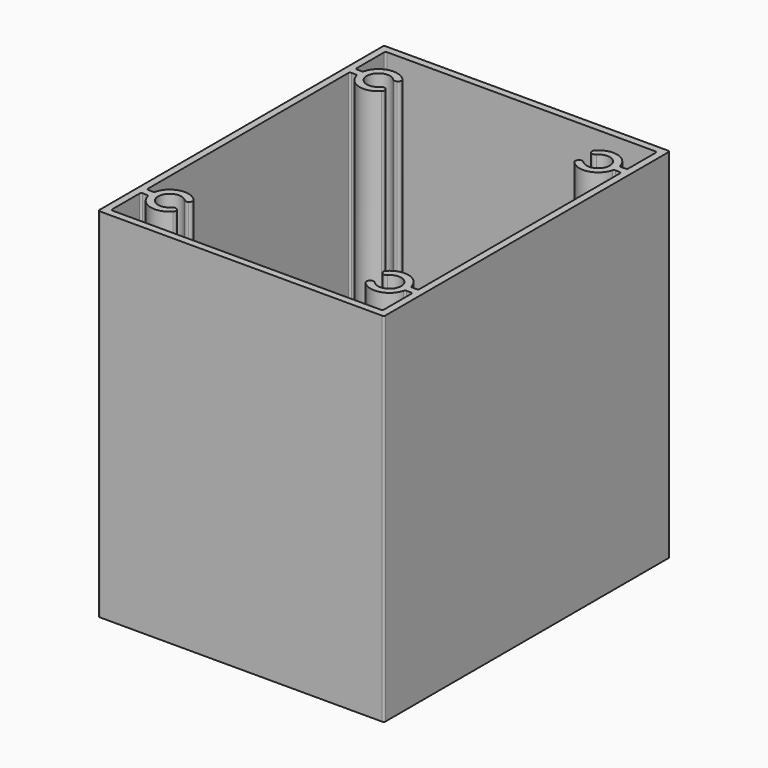
from build123d import *

# Parameters (mm, degrees)
F1_DEPTH = 100


# Not quite as in the source:
# - ends of sketch curves that miss each other by under 0.0002 mm in the source are joined


with BuildPart() as f1:
    # F0 (on Top) → F1 (new body)
    with BuildSketch(Plane.XY):
        with BuildLine():
            Line((40, -49.5), (40, 49.5))
            ThreePointArc((40, 49.5), (39.8535533906, 49.8535533906), (39.5, 50))
            Line((39.5, 50), (-39.5, 50))
            ThreePointArc((-39.5, 50), (-39.8535533906, 49.8535533906), (-40, 49.5))
            Line((-40, 49.5), (-40, -49.5))
            ThreePointArc((-40, -49.5), (-39.8535533906, -49.8535533906), (-39.5, -50))
            Line((-39.5, -50), (39.5, -50))
            ThreePointArc((39.5, -50), (39.8535533906, -49.8535533906), (40, -49.5))
        make_face()
        with BuildLine():
            ThreePointArc((37.5, 48), (37.8535533906, 47.8535533906), (38, 47.5))
            Line((38, 47.5), (38, 38))
            ThreePointArc((38, 38), (37.8535533906, 37.6464466094), (37.5, 37.5))
            Line((37.5, 37.5), (36.300901, 37.5))
            ThreePointArc((36.300901, 37.5), (35.9969413236, 37.6030006107), (35.8182137763, 37.8695659396))
            ThreePointArc((35.8182137763, 37.8695659396), (32.0417405862, 41.5886055318), (26.9486644214, 40.1210975986))
            ThreePointArc((26.9486644214, 40.1210975986), (26.6829406294, 39.2888133915), (27.1727282582, 38.5653394472))
            ThreePointArc((27.1727282582, 38.5653394472), (27.8152796085, 38.4415776294), (28.396791896, 38.7416320991))
            ThreePointArc((28.396791896, 38.7416320991), (34, 36.499999638), (28.3967917139, 34.2583687274))
            ThreePointArc((28.3967917139, 34.2583687274), (27.815279361, 34.5584234062), (27.1727278252, 34.4346613028))
            ThreePointArc((27.1727278252, 34.4346613028), (26.6829405938, 33.711187361), (26.948664104, 32.8789030991))
            ThreePointArc((26.948664104, 32.8789030991), (32.0417407031, 31.4113944979), (35.8182138677, 35.1304350358))
            ThreePointArc((35.8182138677, 35.1304350358), (35.9969417068, 35.3969996827), (36.300901, 35.5))
            Line((36.300901, 35.5), (37.5, 35.5))
            ThreePointArc((37.5, 35.5), (37.8535533906, 35.3535533906), (38, 35))
            Line((38, 35), (38, -35.000003))
            ThreePointArc((38, -35.000003), (37.8535533906, -35.3535563906), (37.5, -35.500003))
            Line((37.5, -35.500003), (36.300901, -35.500003))
            ThreePointArc((36.300901, -35.500003), (35.9969417068, -35.3970026827), (35.8182140282, -35.1304379924))
            ThreePointArc((35.8182140282, -35.1304379924), (32.0417407032, -31.4113974979), (26.948663922, -32.8789059257))
            ThreePointArc((26.948663922, -32.8789059257), (26.6829405938, -33.711190361), (27.1727278252, -34.4346643028))
            ThreePointArc((27.1727278252, -34.4346643028), (27.815279361, -34.5584264062), (28.396791896, -34.2583719009))
            ThreePointArc((28.396791896, -34.2583719009), (34, -36.500002638), (28.3967922133, -38.7416347968))
            ThreePointArc((28.3967922133, -38.7416347968), (27.8152796085, -38.4415806294), (27.1727282582, -38.5653424472))
            ThreePointArc((27.1727282582, -38.5653424472), (26.6829406294, -39.2888163915), (26.948664104, -40.1211009009))
            ThreePointArc((26.948664104, -40.1211009009), (32.0417405862, -41.5886085318), (35.8182136159, -37.8695688962))
            ThreePointArc((35.8182136159, -37.8695688962), (35.9969413236, -37.6030036107), (36.300901, -37.500003))
            Line((36.300901, -37.500003), (37.5, -37.500003))
            ThreePointArc((37.5, -37.500003), (37.8535533906, -37.6464496094), (38, -38.000003))
            Line((38, -38.000003), (38, -47.5))
            ThreePointArc((38, -47.5), (37.8535533906, -47.8535533906), (37.5, -48))
            Line((37.5, -48), (-37.5, -48))
            ThreePointArc((-37.5, -48), (-37.8535533906, -47.8535533906), (-38, -47.5))
            Line((-38, -47.5), (-38, -38.000003))
            ThreePointArc((-38, -38.000003), (-37.8535533906, -37.6464496094), (-37.5, -37.500003))
            Line((-37.5, -37.500003), (-36.300901, -37.500003))
            ThreePointArc((-36.300901, -37.500003), (-35.9969413236, -37.6030036107), (-35.8182137763, -37.8695689396))
            ThreePointArc((-35.8182137763, -37.8695689396), (-32.0417405862, -41.5886085318), (-26.9486644214, -40.1211005986))
            ThreePointArc((-26.9486644214, -40.1211005986), (-26.6829406294, -39.2888163915), (-27.1727282582, -38.5653424472))
            ThreePointArc((-27.1727282582, -38.5653424472), (-27.8152796085, -38.4415806294), (-28.396791896, -38.7416350991))
            ThreePointArc((-28.396791896, -38.7416350991), (-34, -36.500002638), (-28.3967917139, -34.2583717274))
            ThreePointArc((-28.3967917139, -34.2583717274), (-27.815279361, -34.5584264062), (-27.1727278252, -34.4346643028))
            ThreePointArc((-27.1727278252, -34.4346643028), (-26.6829405938, -33.711190361), (-26.948664104, -32.8789060991))
            ThreePointArc((-26.948664104, -32.8789060991), (-32.0417407032, -31.4113974979), (-35.8182138677, -35.1304380358))
            ThreePointArc((-35.8182138677, -35.1304380358), (-35.9969417068, -35.3970026827), (-36.300901, -35.500003))
            Line((-36.300901, -35.500003), (-37.5, -35.500003))
            ThreePointArc((-37.5, -35.500003), (-37.8535533906, -35.3535563906), (-38, -35.000003))
            Line((-38, -35.000003), (-38, 35))
            ThreePointArc((-38, 35), (-37.8535533906, 35.3535533906), (-37.5, 35.5))
            Line((-37.5, 35.5), (-36.300901, 35.5))
            ThreePointArc((-36.300901, 35.5), (-35.9969417068, 35.3969996827), (-35.8182140282, 35.1304349924))
            ThreePointArc((-35.8182140282, 35.1304349924), (-32.0417407031, 31.4113944979), (-26.948663922, 32.8789029257))
            ThreePointArc((-26.948663922, 32.8789029257), (-26.6829405938, 33.711187361), (-27.1727278252, 34.4346613028))
            ThreePointArc((-27.1727278252, 34.4346613028), (-27.815279361, 34.5584234062), (-28.396791896, 34.2583689009))
            ThreePointArc((-28.396791896, 34.2583689009), (-34, 36.499999638), (-28.3967922133, 38.7416317968))
            ThreePointArc((-28.3967922133, 38.7416317968), (-27.8152796085, 38.4415776294), (-27.1727282582, 38.5653394472))
            ThreePointArc((-27.1727282582, 38.5653394472), (-26.6829406294, 39.2888133915), (-26.948664104, 40.1210979009))
            ThreePointArc((-26.948664104, 40.1210979009), (-32.0417405862, 41.5886055318), (-35.8182136159, 37.8695658962))
            ThreePointArc((-35.8182136159, 37.8695658962), (-35.9969413236, 37.6030006107), (-36.300901, 37.5))
            Line((-36.300901, 37.5), (-37.5, 37.5))
            ThreePointArc((-37.5, 37.5), (-37.8535533906, 37.6464466094), (-38, 38))
            Line((-38, 38), (-38, 47.5))
            ThreePointArc((-38, 47.5), (-37.8535533906, 47.8535533906), (-37.5, 48))
            Line((-37.5, 48), (37.5, 48))
        make_face(mode=Mode.SUBTRACT)
    extrude(amount=-F1_DEPTH)


solid = f1.part
